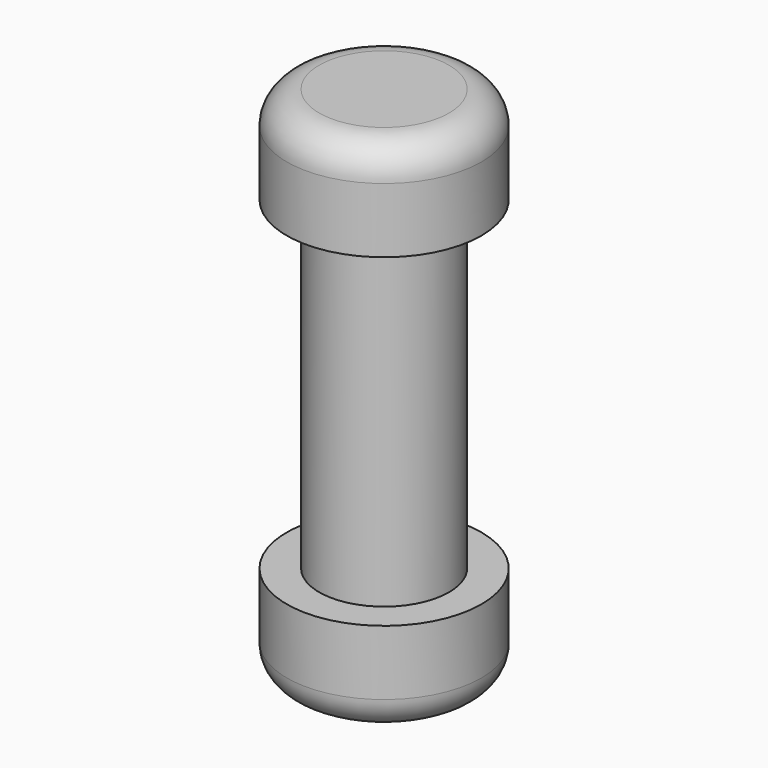
from build123d import *

# Parameters (mm, degrees)
F0_R     = 1
F1_DEPTH = 5
F2_R     = 1.5
F3_DEPTH = 1.5
F4_R     = 0.5
F5_R     = 1.5
F5_R_2   = 1
F6_DEPTH = 1.5
F7_R     = 0.5


with BuildPart() as f1:
    # F0 (on Top) → F1 (new body)
    with BuildSketch(Plane.XY):
        Circle(F0_R)
    extrude(amount=-F1_DEPTH)

    # F2 (on face) → F3 (join)
    with BuildSketch(Plane.XY):
        Circle(F2_R)
    extrude(amount=F3_DEPTH)

    # F4
    f4_edges = [f1.edges().sort_by_distance(p)[0] for p in [
        (-1.5, 0, 1.5),
    ]]
    fillet(f4_edges, radius=F4_R)

    # F5 (on face) → F6 (join)
    with BuildSketch(Plane(origin=(0, 0, -5), x_dir=(1, 0, 0), z_dir=(0, 0, -1))):
        Circle(F5_R)
        Circle(F5_R_2, mode=Mode.SUBTRACT)
        Circle(F5_R_2)
    extrude(amount=F6_DEPTH)

    # F7
    f7_edges = [f1.edges().sort_by_distance(p)[0] for p in [
        (-1.5, 0, -6.5),
    ]]
    fillet(f7_edges, radius=F7_R)


solid = f1.part
